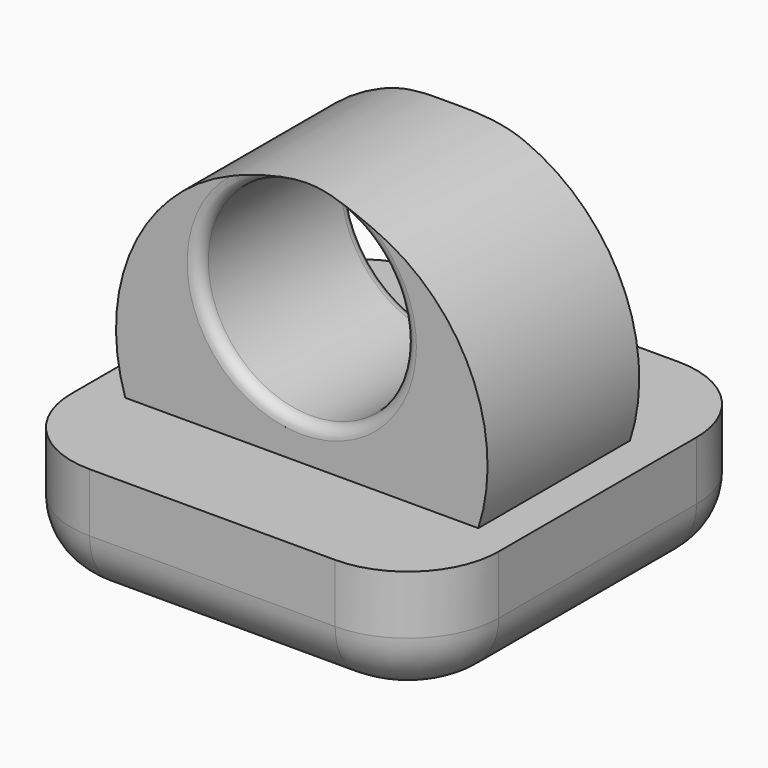
from build123d import *

# Parameters (mm, degrees)
F0_W         = 35.8318164945
F0_H         = 35.9757198021
F1_DEPTH     = 10
F3_R         = 7.62
F4_R         = 5.08
F5_TEXT_SIZE = 10.5716284856
F6_DEPTH     = 3
F2_R         = 8.6263312512
F7_DEPTH     = 15.9


# Not quite as in the source:
# - a fillet or chamfer that OpenCascade refuses, or shapes differently, is made with other operations: its cross-section is extruded or revolved along the edge and cut away or added
# - Text() gives the source's letters only with a copy of the font that has no kerning and outlines rounded to 1/6400 em; it was checked with that copy


with BuildPart() as f1:
    # F0 (on Top) → F1 (new body)
    with BuildSketch(Plane.XY):
        with Locations((-17.9159082472, -7.1951434948)):
            Rectangle(F0_W, F0_H)
    extrude(amount=F1_DEPTH)

    # F3
    f3_edges = [f1.edges().sort_by_distance(p)[0] for p in [
        (-35.831816, -25.183003, 5),
        (-35.831816, 10.792716, 5),
        (0, 10.792716, 5),
        (0, -25.183003, 5),
    ]]
    fillet(f3_edges, radius=F3_R)

    # F4
    f4_edges = [f1.edges().sort_by_distance(p)[0] for p in [
        (-17.915908, -25.183003, 0),
        (-35.831816, -7.195143, 0),
        (-33.59997, -22.951157, 0),
        (-2.231846, -22.951157, 0),
        (0, -7.195143, 0),
        (-2.231846, 8.56087, 0),
        (-17.915908, 10.792716, 0),
        (-33.59997, 8.56087, 0),
    ]]
    fillet(f4_edges, radius=F4_R)

    # F5 (on face) → F6 (cut)
    with BuildSketch(Plane(origin=(0, 0, 0), x_dir=(1, 0, 0), z_dir=(0, 0, -1))):
        with Locations((-30.7518164945, 3.8026284892)):
            Text('bear', F5_TEXT_SIZE, font='Open Sans', text_align=(TextAlign.LEFT, TextAlign.BOTTOM))
    extrude(amount=-F6_DEPTH, mode=Mode.SUBTRACT)


with BuildPart() as f7:
    # F2 (on Front) → F7 (new body)
    with BuildSketch(Plane.XZ):
        with BuildLine():
            ThreePointArc((-3.0451882631, 10.0562060252), (-17.8462229669, 30.4934701062), (-32.6472576708, 10.0562060252))
            Line((-32.6472576708, 10.0562060252), (-29.6020694077, 10.0562060252))
            Line((-29.6020694077, 10.0562060252), (-6.0903765261, 10.0562060252))
            Line((-6.0903765261, 10.0562060252), (-3.0451882631, 10.0562060252))
        make_face()
        with Locations((-17.8462229669, 21.7662632937)):
            Circle(F2_R, mode=Mode.SUBTRACT)
    extrude(amount=F7_DEPTH)

    # F8: fillet of radius 1 on 2 edges, made by hand

    # F8_s1 → F8_t2 (revolve, cut)
    with BuildSketch(Plane.XY.offset(21.7662632937)):
        with BuildLine():
            ThreePointArc((-9.2199917157, -0.9999), (-8.9270984969, -0.2927932188), (-8.2199917157, 0.0001))
            Line((-8.2199917157, 0.0001), (-8.2199917157, 0.0201))
            ThreePointArc((-8.2199917157, 0.0201), (-8.7199417157, 0.02), (-9.2198917157, 0.02))
            Line((-9.2198917157, 0.02), (-9.2398917157, 0))
            ThreePointArc((-9.2398917157, 0), (-9.2398917157, -0.49995), (-9.2399917157, -0.9999))
            Line((-9.2399917157, -0.9999), (-9.2199917157, -0.9999))
        make_face()
    revolve(axis=Axis((-17.8462229669, 0, 21.7662632937), (0, -1, 0)), mode=Mode.SUBTRACT)

    # F8_s3 → F8_t4 (revolve, cut)
    with BuildSketch(Plane.XY.offset(21.7662632937)):
        with BuildLine():
            ThreePointArc((-8.2199917157, -15.9001), (-8.9270984969, -15.6072067812), (-9.2199917157, -14.9001))
            Line((-9.2199917157, -14.9001), (-9.2399917157, -14.9001))
            ThreePointArc((-9.2399917157, -14.9001), (-9.2398917157, -15.40005), (-9.2398917157, -15.9))
            Line((-9.2398917157, -15.9), (-9.2198917157, -15.92))
            ThreePointArc((-9.2198917157, -15.92), (-8.7199417157, -15.92), (-8.2199917157, -15.9201))
            Line((-8.2199917157, -15.9201), (-8.2199917157, -15.9001))
        make_face()
    revolve(axis=Axis((-17.8462229669, -15.9, 21.7662632937), (0, -1, 0)), mode=Mode.SUBTRACT)


solid = Compound([f1.part, f7.part])
